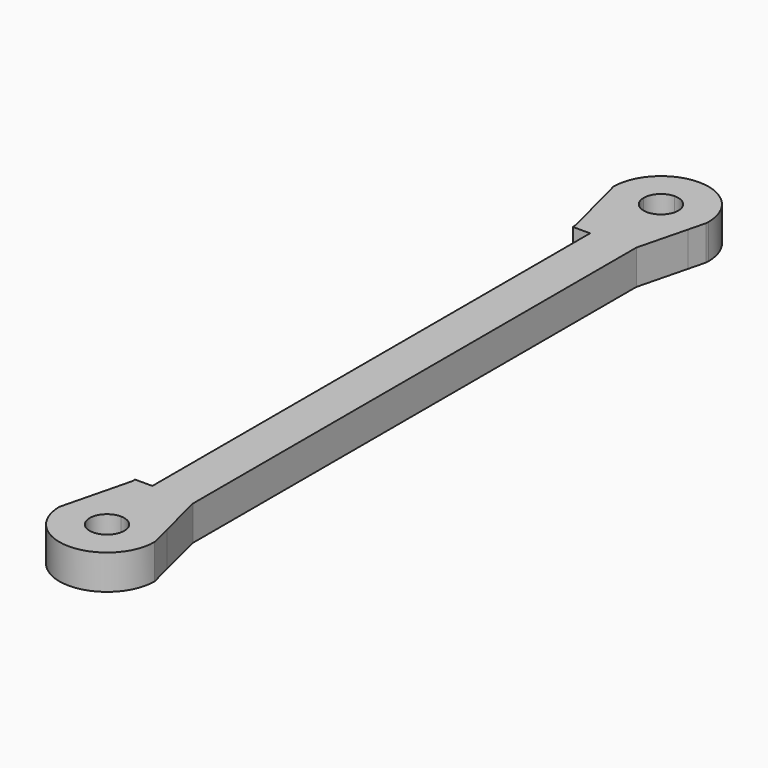
from build123d import *

# Parameters (mm, degrees)
F0_W     = 1.8361258607
F0_H     = 1.0668
F0_W_2   = 7.62
F0_H_2   = 160.4273358566
F1_DEPTH = 10.16
F2_DEPTH = 5.08


with BuildPart() as f1:
    # F0 (on Top) → F1 (new body)
    with BuildSketch(Plane.XY):
        Polygon((6.7189444143, 102.6402935386), (6.7189444143, 103.7061576819), (-2.1710555857, 103.7061576819), (-11.0610555857, 103.7061576819), (-11.0610555857, 102.6402935386), (-5.9810555857, 102.6402935386), (1.6389444143, 102.6402935386), align=None)
        with BuildLine():
            Line((-2.1710555857, 103.7061576819), (6.7189444143, 103.7061576819))
            Line((6.7189444143, 103.7061576819), (10.3688539856, 118.139948899))
            ThreePointArc((10.3688539856, 118.139948899), (5.2686232822, 112.2832362473), (-2.1710555857, 110.0550947226))
            Line((-2.1710555857, 110.0550947226), (-2.1710555857, 103.7061576819))
        make_face()
        with BuildLine():
            Line((-11.0610555857, 103.7061576819), (-2.1710555857, 103.7061576819))
            Line((-2.1710555857, 103.7061576819), (-2.1710555857, 110.0550947226))
            ThreePointArc((-2.1710555857, 110.0550947226), (-9.3601607133, 111.9690507219), (-14.5474187039, 117.301856235))
            Line((-14.5474187039, 117.301856235), (-11.0610555857, 103.7061576819))
        make_face()
        with BuildLine():
            ThreePointArc((-2.1710555857, 110.0550947226), (5.2686232822, 112.2832362473), (10.3688539856, 118.139948899))
            Line((10.3688539856, 118.139948899), (11.6430755059, 123.1789360379))
            ThreePointArc((11.6430755059, 123.1789360379), (11.6622834114, 123.6015178338), (11.668688004, 124.0244874534))
            Line((11.668688004, 124.0244874534), (2.778688004, 124.0244874534))
            ThreePointArc((2.778688004, 124.0244874534), (1.3365515641, 120.4787366559), (-2.1710555857, 118.9461576819))
            Line((-2.1710555857, 118.9461576819), (-2.1710555857, 110.0550947226))
        make_face()
        with Locations((5.8008814839, -58.3204423181)):
            Rectangle(F0_W, F0_H)
        with Locations((-2.1710555857, 22.4266256103)):
            Rectangle(F0_W_2, F0_H_2)
        with BuildLine():
            ThreePointArc((-14.5474187039, 117.301856235), (-9.3601607133, 111.9690507219), (-2.1710555857, 110.0550947226))
            Line((-2.1710555857, 110.0550947226), (-2.1710555857, 118.9461576819))
            ThreePointArc((-2.1710555857, 118.9461576819), (-5.8470627935, 120.3866238933), (-7.381311996, 124.0244874534))
            Line((-7.381311996, 124.0244874534), (-16.271311996, 124.0244874534))
            Line((-16.271311996, 124.0244874534), (-14.5474187039, 117.301856235))
        make_face()
        with BuildLine():
            Line((10.1554150025, -72.599724671), (6.7189444143, -58.8538423181))
            Line((6.7189444143, -58.8538423181), (4.8828185536, -58.8538423181))
            Line((4.8828185536, -58.8538423181), (-2.1710555857, -58.8538423181))
            Line((-2.1710555857, -58.8538423181), (-2.1710555857, -65.2038423181))
            ThreePointArc((-2.1710555857, -65.2038423181), (5.0164501176, -67.1946661459), (10.1554150025, -72.599724671))
        make_face()
        Polygon((4.8828185536, -58.8538423181), (4.8828185536, -57.7870423181), (1.6389444143, -57.7870423181), (-5.9810555857, -57.7870423181), (-11.0610555857, -57.7870423181), (-11.0610555857, -58.8538423181), (-2.1710555857, -58.8538423181), align=None)
        with BuildLine():
            Line((2.778688004, 124.0244874534), (11.668688004, 124.0244874534))
            ThreePointArc((11.668688004, 124.0244874534), (-2.301311996, 137.9944874534), (-16.271311996, 124.0244874534))
            Line((-16.271311996, 124.0244874534), (-7.381311996, 124.0244874534))
            ThreePointArc((-7.381311996, 124.0244874534), (-5.9391755561, 127.5702382509), (-2.4315684063, 129.1028172248))
            ThreePointArc((-2.4315684063, 129.1028172248), (1.2444388015, 127.6623510135), (2.778688004, 124.0244874534))
        make_face()
        with BuildLine():
            Line((11.7989444143, -79.1738423181), (10.1554150025, -72.599724671))
            ThreePointArc((10.1554150025, -72.599724671), (5.0164501176, -67.1946661459), (-2.1710555857, -65.2038423181))
            ThreePointArc((-2.1710555857, -65.2038423181), (-9.3585612891, -67.1946661459), (-14.497526174, -72.599724671))
            Line((-14.497526174, -72.599724671), (-16.1410555857, -79.1738423181))
            ThreePointArc((-16.1410555857, -79.1738423181), (-2.1710555857, -93.1438423181), (11.7989444143, -79.1738423181))
        make_face()
        with BuildLine():
            ThreePointArc((2.9089444143, -79.1738423181), (-5.7631580342, -82.7659447665), (-2.1710555857, -74.0938423181))
            ThreePointArc((-2.1710555857, -74.0938423181), (1.4210468627, -75.5817398696), (2.9089444143, -79.1738423181))
        make_face(mode=Mode.SUBTRACT)
        with BuildLine():
            Line((-2.1710555857, -65.2038423181), (-2.1710555857, -58.8538423181))
            Line((-2.1710555857, -58.8538423181), (-11.0610555857, -58.8538423181))
            Line((-11.0610555857, -58.8538423181), (-14.497526174, -72.599724671))
            ThreePointArc((-14.497526174, -72.599724671), (-9.3585612891, -67.1946661459), (-2.1710555857, -65.2038423181))
        make_face()
    extrude(amount=F1_DEPTH)

    # F2 (add): a face of the model
    f2_faces = [f1.faces().sort_by_distance(p)[0] for p in [
        (1.6389444143, 22.4266256103, 5.08),
    ]]
    extrude(f2_faces, amount=F2_DEPTH)


solid = f1.part
